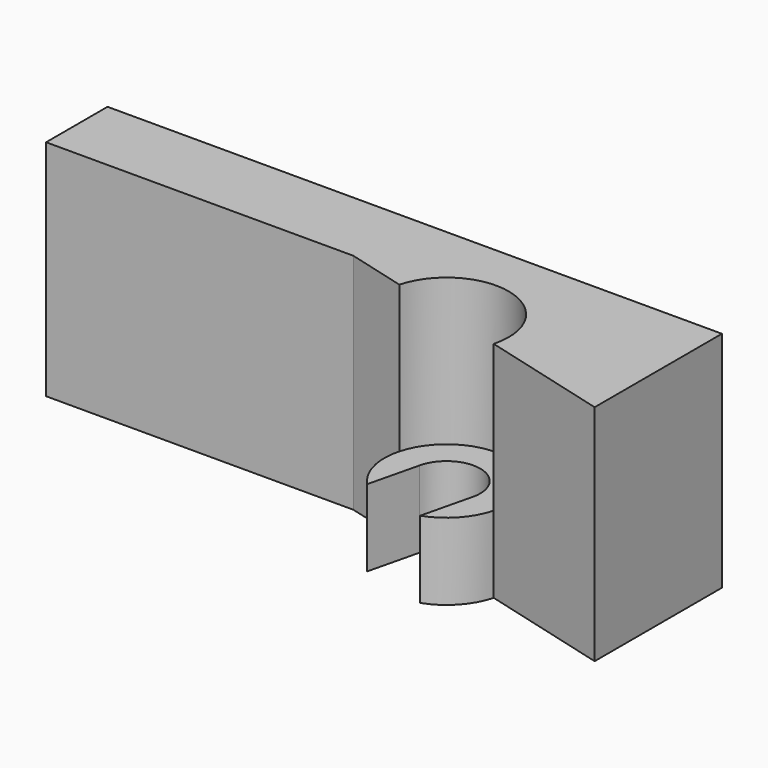
from build123d import *

# Parameters (mm, degrees)
F1_DEPTH  = 25.4
F3_DEPTH  = 152.4
F4_R      = 5.1395
F5_DEPTH  = 152.401
F7_DEPTH  = 6.096
F9_DEPTH  = 6.35
F10_R     = 1.905
F11_DEPTH = 6.35
F12_W     = 46.7241909355
F12_H     = 189.791161567
F13_DEPTH = 50.801


with BuildPart() as f1:
    # F0 (on Right) → F1 (new body)
    with BuildSketch(Plane.YZ):
        Polygon((-6.35, 0), (0, 0), (0, 203.2), (-24.13, 203.2), (-24.13, 177.8), (-17.78, 177.8), (-17.78, 196.85), (-6.35, 196.85), align=None)
    extrude(amount=F1_DEPTH)

    # F2 (on Top) → F3 (join)
    with BuildSketch(Plane.XY):
        Polygon((50.8, 0), (25.4, 0), (25.4, -6.35), (50.8, -13.1559094878), align=None)
    extrude(amount=F3_DEPTH)

    # F4 (on face) → F5 (cut, through all)
    with BuildSketch(Plane.XY.offset(152.4)):
        with Locations((35.2138063951, -8.9796014982)):
            Circle(F4_R)
    extrude(amount=-F5_DEPTH, mode=Mode.SUBTRACT)

    # F6 (on face) → F7 (cut)
    with BuildSketch(Plane.YZ.offset(50.8)):
        Polygon((-9.3719547439, 71.3606500437), (-3.7839547439, 71.3606500437), (-0.9899547439, 76.2), (-3.7839547439, 81.0393499563), (-9.3719547439, 81.0393499563), (-12.1659547439, 76.2), align=None)
    extrude(amount=-F7_DEPTH, mode=Mode.SUBTRACT)

    # F8 (on face) → F9 (join)
    with BuildSketch(Plane(origin=(0, 0, 0), x_dir=(1, 0, 0), z_dir=(0, 0, -1))):
        with BuildLine():
            Line((32.4918402484, 8.3672288206), (31.4877265179, 12.5194869482))
            ThreePointArc((31.4877265179, 12.5194869482), (30.2327985505, 10.2461010452), (30.2494306109, 7.6494010159))
            ThreePointArc((30.2494306109, 7.6494010159), (36.5440068774, 4.015225714), (40.1781821793, 10.3098019805))
            ThreePointArc((40.1781821793, 10.3098019805), (38.9811201217, 12.4755716834), (36.9107028801, 13.8308902517))
            Line((36.9107028801, 13.8308902517), (37.9148166106, 9.678632124))
            ThreePointArc((37.9148166106, 9.678632124), (37.9256407477, 9.6353868624), (37.9357725418, 9.5919741759))
            ThreePointArc((37.9357725418, 9.5919741759), (35.8261790728, 6.2576353516), (32.4918402484, 8.3672288206))
        make_face()
    extrude(amount=-F9_DEPTH)

    # F10 (on face) → F11 (join)
    with BuildSketch(Plane(origin=(0.1139773719, 0.425369343, 0), x_dir=(0.9659258263, -0.2588190451, 0), z_dir=(-0.2588190451, -0.9659258263, 0))):
        with Locations((45.3620319066, 149.352)):
            Circle(F10_R)
        with Locations((49.4260319066, 145.288)):
            Circle(F10_R)
    extrude(amount=F11_DEPTH)

    # F12 (on face) → F13 (cut, through all)
    with BuildSketch(Plane.YZ.offset(50.8)):
        with Locations((-7.7233714983, 113.3844163269)):
            Rectangle(F12_W, F12_H)
    extrude(amount=-F13_DEPTH, mode=Mode.SUBTRACT)


solid = f1.part
